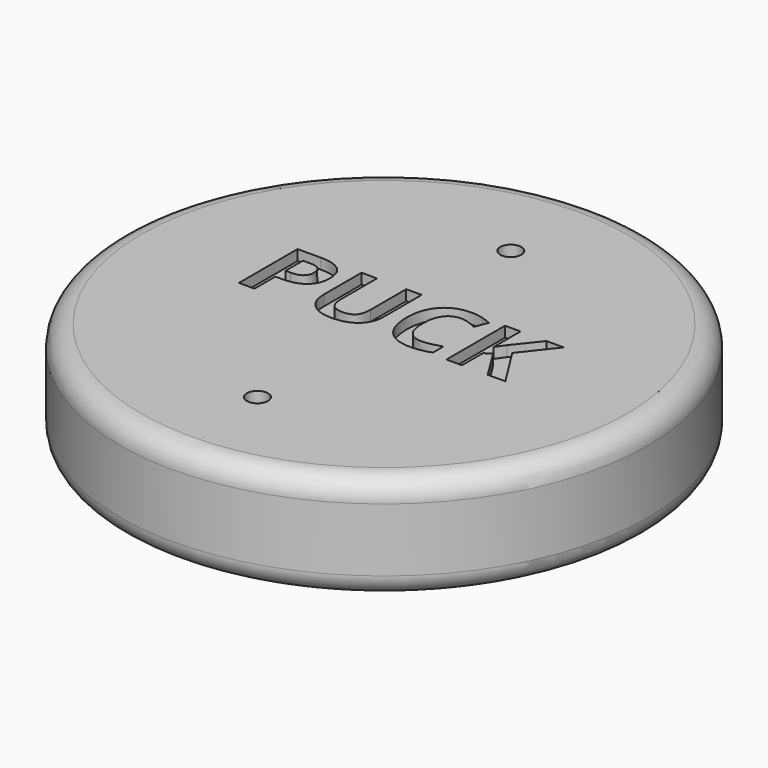
from build123d import *

# Parameters (mm, degrees)
F0_R           = 25
F1_DEPTH       = 10
F2_TEXT_SIZE   = 9.7222222222
F3_DEPTH       = 1
F4_R           = 2
F6_D           = 2
F6_CBORE_D     = 5
F6_CBORE_DEPTH = 2.5


# Not quite as in the source:
# - Text() gives the source's letters only with a copy of the font that has no kerning and outlines rounded to 1/6400 em; it was checked with that copy


with BuildPart() as f1:
    # F0 (on Top) → F1 (new body)
    with BuildSketch(Plane.XY):
        Circle(F0_R)
    extrude(amount=F1_DEPTH)

    # F2 (on face) → F3 (cut)
    with BuildSketch(Plane.XY.offset(10)):
        with Locations((-13.3680555556, -1.5653021657)):
            Text('PUCK', F2_TEXT_SIZE, font='Open Sans', font_style=FontStyle.BOLD, text_align=(TextAlign.LEFT, TextAlign.BOTTOM))
    extrude(amount=-F3_DEPTH, mode=Mode.SUBTRACT)

    # F4
    f4_edges = [f1.edges().sort_by_distance(p)[0] for p in [
        (-25, 0, 10),
        (-25, 0, 0),
    ]]
    fillet(f4_edges, radius=F4_R)

    # F6 (through all)
    with Locations(Plane(origin=(0, 0, 0), x_dir=(1, 0, 0), z_dir=(0, 0, -1))):
        with Locations((0, 15), (0, -15)):
            CounterBoreHole(F6_D / 2, F6_CBORE_D / 2, F6_CBORE_DEPTH)


solid = f1.part
